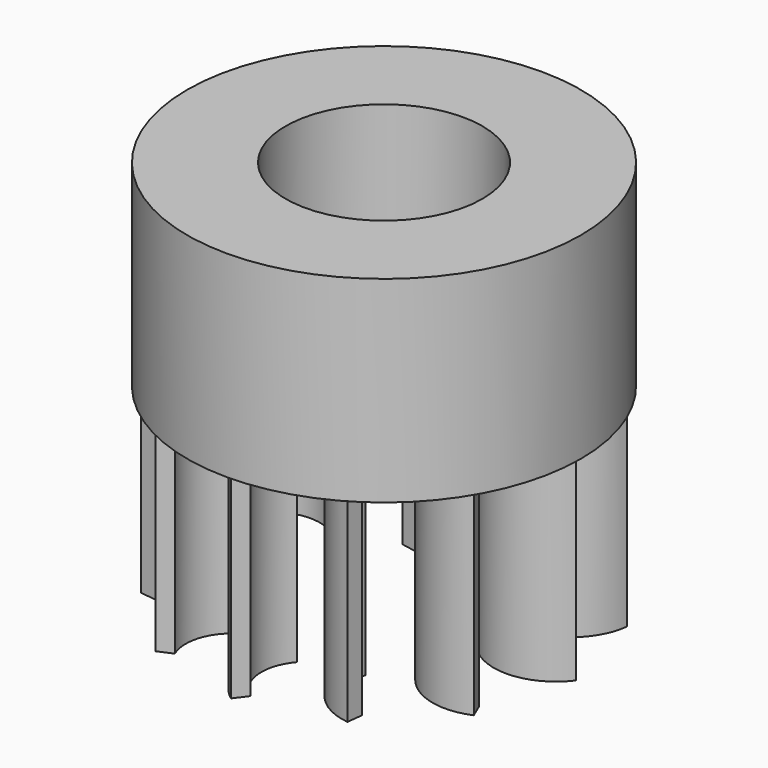
from build123d import *

# Parameters (mm, degrees)
F0_R            = 50
F1_DEPTH        = 50
F2_R            = 25
F3_DEPTH        = 50
F5_DEPTH        = 50
F5_COPIES_COUNT = 12


# Not quite as in the source:
# - a pattern or mirror of a feature is missing from the dataset's text; its kind, count and spacing are read off the source's solid


with BuildPart() as f1:
    # F0 (on Top) → F1 (new body)
    with BuildSketch(Plane.XY):
        Circle(F0_R)
    extrude(amount=F1_DEPTH)

    # F2 (on Top) → F3 (cut)
    with BuildSketch(Plane.XY):
        Circle(F2_R)
    extrude(amount=F3_DEPTH, mode=Mode.SUBTRACT)

    # F4 (on Top) → F5 (join)
    with BuildSketch(Plane.XY):
        with BuildLine():
            Line((24.2363690546, 14.6788293603), (23.4842319041, 10.750179179))
            ThreePointArc((23.4842319041, 10.750179179), (35.7966783621, 13.5258846201), (42.1475842595, 24.4330782443))
            Line((42.1475842595, 24.4330782443), (38.1746449562, 24.8975734892))
            ThreePointArc((38.1746449562, 24.8975734892), (33.4316236094, 16.7517982205), (24.2363690546, 14.6788293603))
        make_face()
    f5 = extrude(amount=-F5_DEPTH)

    # F5_copies: F5 ×12 about axis
    f5_copies_axis = Axis((0, 0, 0), (0, 0, 1))
    for i in range(1, F5_COPIES_COUNT):
        add(f5.rotate(f5_copies_axis, i * 360 / F5_COPIES_COUNT))


solid = f1.part
